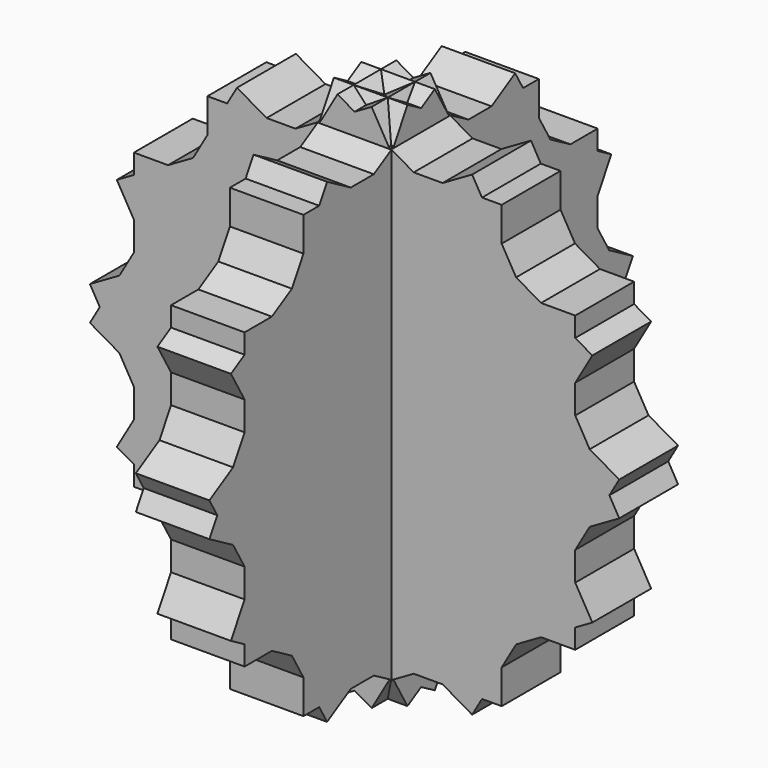
from build123d import *

# Parameters (mm, degrees)
F1_DEPTH = 5
F2_COUNT = 12
F4_DEPTH = 5
F5_COUNT = 12


with BuildPart() as f1:
    # F0 (on Front) → F1 (new body, symmetric)
    with BuildSketch(Plane.XZ):
        with BuildLine():
            Line((-30, 0), (0, 0))
            Line((0, 0), (0, 20))
            ThreePointArc((0, 20), (-17.5, 22.5), (-15, 40))
            Line((-15, 40), (-30, 40))
            Line((-30, 40), (-30, 0))
        make_face()
    extrude(amount=F1_DEPTH, both=True)

    # F2: F1 ×12 about axis
    f2_axis = Axis((0, 0, 20), (0, 1, 0))


with BuildPart() as f1_1:
    add(f1.part)
    for i in range(1, F2_COUNT):
        add(f1.part.rotate(f2_axis, i * 360 / F2_COUNT))


with BuildPart() as f4:
    # F3 (on Right) → F4 (new body, symmetric)
    with BuildSketch(Plane.YZ):
        with BuildLine():
            Line((-29.9398601055, 0), (0.0601398945, 0))
            Line((0.0601398945, 0), (0.0601398945, 20))
            ThreePointArc((0.0601398945, 20), (-17.4398601055, 22.5), (-14.9398601055, 40))
            Line((-14.9398601055, 40), (-29.9398601055, 40))
            Line((-29.9398601055, 40), (-29.9398601055, 0))
        make_face()
    extrude(amount=F4_DEPTH, both=True)

    # F5: F4 ×12 about axis
    f5_axis = Axis((0, 0.0601398945, 20), (-1, 0, 0))


with BuildPart() as f4_1:
    add(f4.part)
    for i in range(1, F5_COUNT):
        add(f4.part.rotate(f5_axis, i * 360 / F5_COUNT))


solid = Compound([f1_1.part, f4_1.part])
